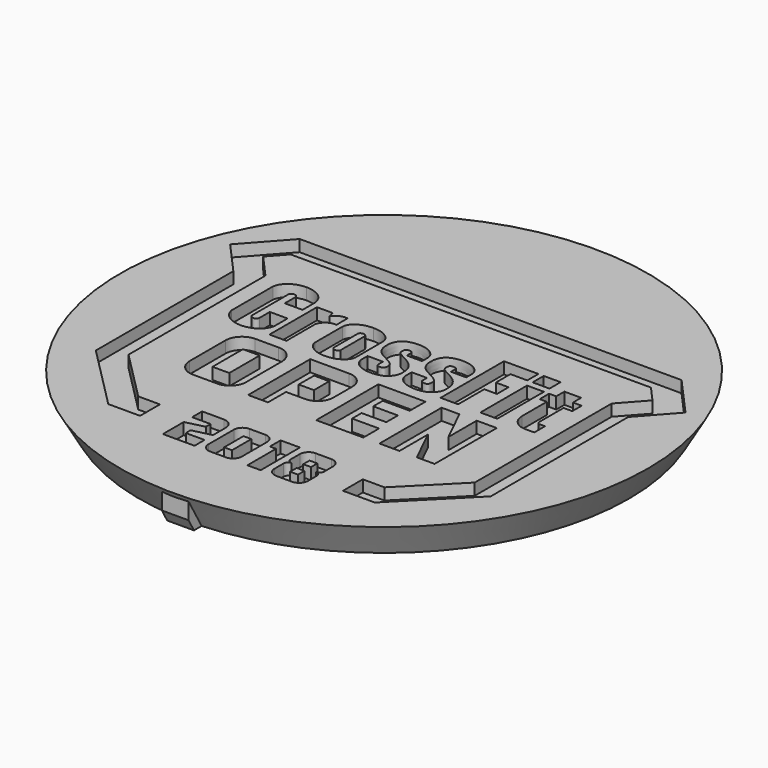
from build123d import *

# Parameters (mm, degrees)
F0_R        = 28.956
F1_DEPTH    = 3.556
F2_W        = 30.4023699468
F2_H        = 2.708328606
F2_W_2      = 1.8437616527
F2_H_2      = 6.3712084666
F2_H_3      = 1.5175901353
F2_W_3      = 1.6611122992
F2_H_4      = 2.0968401222
F2_W_4      = 1.8359664828
F2_H_5      = 4.1484234825
F2_W_5      = 0.8592136437
F2_H_6      = 2.6414245367
F2_H_7      = 0.8889122684
F2_H_8      = 0.8636
F3_DEPTH    = 1.27
F6_DEPTH    = 3.556
F7_T1_DEPTH = 9.4921978168


# Not quite as in the source:
# - a fillet or chamfer that OpenCascade refuses, or shapes differently, is made with other operations: its cross-section is extruded or revolved along the edge and cut away or added


with BuildPart() as f1:
    # F0 (on Top) → F1 (new body)
    with BuildSketch(Plane.XY):
        Circle(F0_R)
    extrude(amount=F1_DEPTH)

    # F2 (on face) → F3 (cut)
    with BuildSketch(Plane.XY.offset(3.556)):
        with Locations((0, 13.1786047998)):
            Rectangle(F2_W, F2_H)
        Polygon((20.8420716974, 14.5327691028), (15.2011849734, 14.5327691028), (15.2011849734, 11.8244404968), (19.6655910583, 11.8244404968), (21.247090707, 10.0590654712), (18.8943144933, 7.4307704384), (18.8943144933, -11.2499324565), (13.4406701729, -16.7418979069), (11.0729235041, -16.7418979069), (11.0729235041, -19.4502265129), (14.5413199249, -19.4502265129), (21.5503721796, -12.3919237413), (21.5503721796, 6.3732514918), (24.849809781, 10.0590654712), align=None)
        Polygon((-15.2011849734, 11.8244404968), (-15.2011849734, 14.5327691028), (-20.8420716974, 14.5327691028), (-24.849809781, 10.0590654712), (-21.5503721796, 6.3732514918), (-21.5503721796, -12.3919237413), (-14.5413199249, -19.4502265129), (-11.0729235041, -19.4502265129), (-11.0729235041, -16.7418979069), (-13.4406701729, -16.7418979069), (-18.8943144933, -11.2499324565), (-18.8943144933, 7.4307704384), (-21.247090707, 10.0590654712), (-19.6655910583, 11.8244404968), align=None)
        with BuildLine():
            ThreePointArc((-15.2091418535, 6.0097032957), (-14.8139919296, 6.2693332665), (-14.4188420058, 6.0097032957))
            Line((-14.4188420058, 6.0097032957), (-14.4188420058, 4.4719388507))
            Line((-14.4188420058, 4.4719388507), (-12.4801692695, 4.4719388507))
            Line((-12.4801692695, 4.4719388507), (-12.4801692695, 6.2930637769))
            add(Edge.make_bspline(
                [(-12.4801692695, 6.2930637769), (-12.5916933403, 6.7707157481), (-12.9251884268, 7.2707731335), (-13.6344023128, 7.7464624472), (-14.2989607428, 7.9362339904), (-14.8139919296, 7.9558056579)],
                knots=[0, 0, 0, 0, 0.3452518733, 0.6338422719, 1, 1, 1, 1], degree=3))
            add(Edge.make_bspline(
                [(-17.1478145898, 6.2930637769), (-17.036290519, 6.7707157481), (-16.7027954325, 7.2707731335), (-15.9935815465, 7.7464624472), (-15.3290231165, 7.9362339904), (-14.8139919296, 7.9558056579)],
                knots=[0, 0, 0, 0, 0.3452518733, 0.6338422719, 1, 1, 1, 1], degree=3))
            Line((-17.1478145898, 6.2930637769), (-17.1478145898, 0.6190669056))
            add(Edge.make_bspline(
                [(-17.1478145898, 0.6190669056), (-17.036290519, 0.1414149345), (-16.7027954325, -0.3586424509), (-15.9935815465, -0.8343317647), (-15.3290231165, -1.0241033079), (-14.8139919296, -1.0436749754)],
                knots=[0, 0, 0, 0, 0.3452518733, 0.6338422719, 1, 1, 1, 1], degree=3))
            add(Edge.make_bspline(
                [(-12.4801692695, 0.6190669056), (-12.5916933403, 0.1414149345), (-12.9251884268, -0.3586424509), (-13.6344023128, -0.8343317647), (-14.2989607428, -1.0241033079), (-14.8139919296, -1.0436749754)],
                knots=[0, 0, 0, 0, 0.3452518733, 0.6338422719, 1, 1, 1, 1], degree=3))
            Line((-12.4801692695, 0.6190669056), (-12.4801692695, 2.4332190197))
            Line((-12.4801692695, 2.4332190197), (-14.4188420058, 2.4332190197))
            Line((-14.4188420058, 2.4332190197), (-14.4188420058, 1.0003426842))
            ThreePointArc((-14.4188420058, 1.0003426842), (-14.8139919296, 0.6797582705), (-15.2091418535, 1.0003426842))
            Line((-15.2091418535, 1.0003426842), (-15.2091418535, 6.0097032957))
        make_face()
        with BuildLine():
            ThreePointArc((-8.498294748, 5.6527445823), (-9.3240459461, 5.52802916), (-9.9700721946, 4.9988136426))
            Line((-9.9700721946, 4.9988136426), (-10.0917066481, 5.6280705877))
            Line((-10.0917066481, 5.6280705877), (-11.8310791474, 5.6280705877))
            Line((-11.8310791474, 5.6280705877), (-11.8310791474, -0.8495571991))
            Line((-11.8310791474, -0.8495571991), (-9.9822352674, -0.8495571991))
            Line((-9.9822352674, -0.8495571991), (-9.9822352674, 3.0987069741))
            ThreePointArc((-9.9822352674, 3.0987069741), (-9.4355214126, 3.8909649876), (-8.498294748, 4.1104529783))
            Line((-8.498294748, 4.1104529783), (-8.498294748, 5.6527445823))
        make_face()
        with BuildLine():
            add(Edge.make_bspline(
                [(-7.8876619975, 4.1982766971), (-7.8356496049, 4.6341372871), (-7.4830251688, 5.0855806361), (-6.6969666534, 5.5265744778), (-6.1764580028, 5.6217318842), (-5.6770178073, 5.6407110794)],
                knots=[0, 0, 0, 0, 0.3397100712, 0.6449265753, 1, 1, 1, 1], degree=3))
            Line((-7.8876619975, 4.1982766971), (-7.8876619975, 0.4633077452))
            add(Edge.make_bspline(
                [(-7.8876619975, 0.4633077452), (-7.8356496049, 0.0274471552), (-7.4830251688, -0.4239961938), (-6.6969666534, -0.8649900355), (-6.1764580028, -0.9601474419), (-5.6770178073, -0.9791266371)],
                knots=[0, 0, 0, 0, 0.3397100712, 0.6449265753, 1, 1, 1, 1], degree=3))
            add(Edge.make_bspline(
                [(-3.4663736171, 0.4633077452), (-3.5183860098, 0.0274471552), (-3.8710104458, -0.4239961938), (-4.6570689612, -0.8649900355), (-5.1775776118, -0.9601474419), (-5.6770178073, -0.9791266371)],
                knots=[0, 0, 0, 0, 0.3397100712, 0.6449265753, 1, 1, 1, 1], degree=3))
            Line((-3.4663736171, 0.4633077452), (-3.4663736171, 4.1982766971))
            add(Edge.make_bspline(
                [(-3.4663736171, 4.1982766971), (-3.5183860098, 4.6341372871), (-3.8710104458, 5.0855806361), (-4.6570689612, 5.5265744778), (-5.1775776118, 5.6217318842), (-5.6770178073, 5.6407110794)],
                knots=[0, 0, 0, 0, 0.3397100712, 0.6449265753, 1, 1, 1, 1], degree=3))
        make_face()
        with BuildLine():
            Line((-6.0537514093, 0.6796154458), (-6.0537514093, 4.0396556988))
            ThreePointArc((-6.0537514093, 4.0396556988), (-5.6770178073, 4.2767262399), (-5.3002842053, 4.0396556988))
            Line((-5.3002842053, 4.0396556988), (-5.3002842053, 0.6796154458))
            ThreePointArc((-5.3002842053, 0.6796154458), (-5.6770178073, 0.4325808427), (-6.0537514093, 0.6796154458))
        make_face(mode=Mode.SUBTRACT)
        with BuildLine():
            add(Edge.make_bspline(
                [(-2.8303159575, 0.3884340668), (-2.8039437057, 0.2035950511), (-2.7084645464, -0.0700189873), (-2.3608920836, -0.4703230086), (-1.9926629718, -0.6996264871), (-1.5028929662, -0.8748491288), (-1.0382407316, -0.9538686812), (-0.6882680471, -0.9546334772), (-0.3368604514, -0.9540527619), (0.2211413136, -0.8513074189), (0.612300795, -0.6901154246), (0.9801185549, -0.3981460143), (1.2267344248, -0.0690546676), (1.3993589582, 0.2977634954), (1.4223729478, 0.7584350911), (1.4049419285, 1.1135593111), (1.3286013981, 1.553696764), (1.1223334914, 1.9521079504), (0.8760135922, 2.2676339155), (0.6015247761, 2.5058684812), (0.2906951276, 2.7053452538), (-0.0001070692, 2.8824823952), (-0.3353974242, 3.0432490404), (-0.5764466432, 3.1792562527), (-0.8154579768, 3.303817088), (-0.9633304165, 3.4276750313), (-1.0959908548, 3.6333141563), (-1.0823984853, 3.8622415727), (-1.0834469924, 4.0754389156), (-0.9485709412, 4.2583690073), (-0.7487440326, 4.3029808765), (-0.5601470729, 4.2949903255), (-0.3773783712, 4.2385764575), (-0.3052749299, 4.1735809243), (-0.2735022713, 4.0681006186)],
                knots=[0, 0, 0, 0, 0.0370250499, 0.0748342879, 0.1100620625, 0.1484988784, 0.1852224027, 0.2162968341, 0.2479903621, 0.2879321478, 0.3230237776, 0.3590762656, 0.3932110531, 0.4269990648, 0.4628119337, 0.4948648069, 0.530192635, 0.5659957163, 0.5996315799, 0.6317213982, 0.6639857771, 0.6953892736, 0.7277821278, 0.7561961656, 0.7835044746, 0.8069782815, 0.8326158776, 0.857980682, 0.8824603672, 0.9067304417, 0.9303429697, 0.953652975, 0.975833924, 1, 1, 1, 1], degree=3))
            Line((-0.2735022713, 4.0681006186), (-0.2735022713, 3.4427449837))
            Line((-0.2735022713, 3.4427449837), (1.3895077923, 3.4427449837))
            Line((1.3895077923, 3.4427449837), (1.3895077923, 4.2547744498))
            add(Edge.make_bspline(
                [(1.3895077923, 4.2547744498), (1.362871865, 4.4414615263), (1.2883734828, 4.7378016949), (0.9605026276, 5.0998324979), (0.5716220009, 5.3815223969), (0.0152610688, 5.5827557819), (-0.3948809767, 5.6297560073), (-0.7047527982, 5.6499225931), (-1.0751777633, 5.6320466323), (-1.6282857111, 5.5504935604), (-2.0336875884, 5.3727640469), (-2.4117723458, 5.0855965451), (-2.6319171142, 4.7457920238), (-2.777638503, 4.3159693257), (-2.7948365878, 3.9652673217), (-2.7867872003, 3.5566089511), (-2.7234512303, 3.1492983197), (-2.4809077804, 2.7167962496), (-2.2560062896, 2.466619706), (-1.9772894721, 2.263975186), (-1.613083499, 2.067015106), (-1.2952433521, 1.9125631017), (-1.0179124703, 1.7567271658), (-0.7490698208, 1.6103729622), (-0.506207899, 1.4077450313), (-0.4071682892, 1.2885965948), (-0.2936071786, 1.0792376552), (-0.3010610885, 0.7910872402), (-0.3213241393, 0.5663172014), (-0.4513056845, 0.4078239751), (-0.6386646385, 0.3709036814), (-0.8427860612, 0.3772912723), (-1.0484772467, 0.4306358217), (-1.1223962588, 0.5223560412), (-1.1560394719, 0.6340462979)],
                knots=[0, 0, 0, 0, 0.0373952344, 0.0734858494, 0.1105806222, 0.1514081281, 0.1855398741, 0.2145930161, 0.246989669, 0.2866513485, 0.3223486125, 0.3583549464, 0.3922575872, 0.4276388924, 0.4592443755, 0.4928782518, 0.5272671439, 0.5643692779, 0.5951310751, 0.6260952205, 0.6604130771, 0.6921960524, 0.7219608284, 0.7518311519, 0.7813056856, 0.8022259164, 0.8274762943, 0.8561110411, 0.8813007038, 0.9041610683, 0.9268832448, 0.9511148768, 0.9744111926, 1, 1, 1, 1], degree=3))
            Line((-1.1560394719, 0.6340462979), (-1.1560394719, 1.2829401795))
            Line((-1.1560394719, 1.2829401795), (-2.8303159575, 1.2829401795))
            Line((-2.8303159575, 1.2829401795), (-2.8303159575, 0.3884340668))
        make_face()
        with BuildLine():
            add(Edge.make_bspline(
                [(1.9797450798, 0.3972758105), (2.0061173315, 0.2124367948), (2.1015964908, -0.0611772436), (2.4491689536, -0.4614812649), (2.8173980654, -0.6907847434), (3.307168071, -0.8660073851), (3.7718203056, -0.9450269375), (4.1217929901, -0.9457917335), (4.4732005858, -0.9452110182), (5.0312023509, -0.8424656752), (5.4223618323, -0.6812736809), (5.7901795921, -0.3893042706), (6.036795462, -0.0602129239), (6.2094199954, 0.3066052391), (6.232433985, 0.7672768348), (6.2150029657, 1.1224010548), (6.1386624353, 1.5625385077), (5.9323945286, 1.9609496941), (5.6860746294, 2.2764756592), (5.4115858133, 2.5147102249), (5.1007561648, 2.7141869975), (4.809953968, 2.8913241389), (4.474663613, 3.0520907841), (4.233614394, 3.1880979964), (3.9946030604, 3.3126588317), (3.8467306207, 3.436516775), (3.7140701824, 3.6421559), (3.7276625519, 3.8710833164), (3.7266140448, 4.0842806593), (3.861490096, 4.267210751), (4.0613170047, 4.3118226202), (4.2499139643, 4.3038320692), (4.4326826661, 4.2474182012), (4.5047861073, 4.182422668), (4.5365587659, 4.0769423623)],
                knots=[0, 0, 0, 0, 0.0370250499, 0.0748342879, 0.1100620625, 0.1484988784, 0.1852224027, 0.2162968341, 0.2479903621, 0.2879321478, 0.3230237776, 0.3590762656, 0.3932110531, 0.4269990648, 0.4628119337, 0.4948648069, 0.530192635, 0.5659957163, 0.5996315799, 0.6317213982, 0.6639857771, 0.6953892736, 0.7277821278, 0.7561961656, 0.7835044746, 0.8069782815, 0.8326158776, 0.857980682, 0.8824603672, 0.9067304417, 0.9303429697, 0.953652975, 0.975833924, 1, 1, 1, 1], degree=3))
            Line((4.5365587659, 4.0769423623), (4.5365587659, 3.4515867274))
            Line((4.5365587659, 3.4515867274), (6.1995688295, 3.4515867274))
            Line((6.1995688295, 3.4515867274), (6.1995688295, 4.2636161935))
            add(Edge.make_bspline(
                [(6.1995688295, 4.2636161935), (6.1729329022, 4.45030327), (6.09843452, 4.7466434386), (5.7705636648, 5.1086742416), (5.3816830381, 5.3903641406), (4.825322106, 5.5915975256), (4.4151800605, 5.638597751), (4.105308239, 5.6587643368), (3.7348832739, 5.640888376), (3.1817753261, 5.5593353041), (2.7763734488, 5.3816057906), (2.3982886914, 5.0944382888), (2.178143923, 4.7546337675), (2.0324225342, 4.3248110694), (2.0152244495, 3.9741090653), (2.0232738369, 3.5654506948), (2.0866098069, 3.1581400634), (2.3291532568, 2.7256379933), (2.5540547477, 2.4754614497), (2.8327715651, 2.2728169297), (3.1969775382, 2.0758568497), (3.5148176851, 1.9214048454), (3.7921485669, 1.7655689095), (4.0609912164, 1.6192147059), (4.3038531382, 1.416586775), (4.402892748, 1.2974383385), (4.5164538586, 1.0880793989), (4.5089999487, 0.7999289839), (4.4887368979, 0.5751589451), (4.3587553528, 0.4166657188), (4.1713963987, 0.3797454251), (3.967274976, 0.386133016), (3.7615837905, 0.4394775654), (3.6876647784, 0.5311977848), (3.6540215653, 0.6428880416)],
                knots=[0, 0, 0, 0, 0.0373952344, 0.0734858494, 0.1105806222, 0.1514081281, 0.1855398741, 0.2145930161, 0.246989669, 0.2866513485, 0.3223486125, 0.3583549464, 0.3922575872, 0.4276388924, 0.4592443755, 0.4928782518, 0.5272671439, 0.5643692779, 0.5951310751, 0.6260952205, 0.6604130771, 0.6921960524, 0.7219608284, 0.7518311519, 0.7813056856, 0.8022259164, 0.8274762943, 0.8561110411, 0.8813007038, 0.9041610683, 0.9268832448, 0.9511148768, 0.9744111926, 1, 1, 1, 1], degree=3))
            Line((3.6540215653, 0.6428880416), (3.6540215653, 1.2917819232))
            Line((3.6540215653, 1.2917819232), (1.9797450798, 1.2917819232))
            Line((1.9797450798, 1.2917819232), (1.9797450798, 0.3972758105))
        make_face()
        Polygon((10.6105204249, 6.2751232445), (10.6105204249, 7.7927133799), (6.8492461505, 7.7927133799), (6.8492461505, -0.854884015), (8.7667587722, -0.854884015), (8.7667587722, 2.7055770889), (10.1574822838, 2.7055770889), (10.1574822838, 4.2872906461), (8.7667587722, 4.2872906461), (8.7667587722, 6.2751232445), align=None)
        with Locations((12.1124403237, 2.3307202183)):
            Rectangle(F2_W_2, F2_H_2)
        with Locations((12.1124403237, 7.0339183122)):
            Rectangle(F2_W_2, F2_H_3)
        with BuildLine():
            Line((16.2016264889, 6.6334225968), (14.3765285406, 6.6334225968))
            Line((14.3765285406, 6.6334225968), (14.3765285406, 5.5163244516))
            Line((14.3765285406, 5.5163244516), (13.5945966262, 5.5163244516))
            Line((13.5945966262, 5.5163244516), (13.5945966262, 4.2304804347))
            Line((13.5945966262, 4.2304804347), (14.3765285406, 4.2304804347))
            Line((14.3765285406, 4.2304804347), (14.3765285406, 0.8540854588))
            ThreePointArc((14.3765285406, 0.8540854588), (14.8770741106, -0.354338445), (16.0854980144, -0.854884015))
            Line((16.0854980144, -0.854884015), (17.0765723828, -0.854884015))
            Line((17.0765723828, -0.854884015), (17.0765723828, 0.6118975844))
            Line((17.0765723828, 0.6118975844), (16.5136363152, 0.6118975844))
            ThreePointArc((16.5136363152, 0.6118975844), (16.2930120512, 0.7032831468), (16.2016264889, 0.9239074107))
            Line((16.2016264889, 0.9239074107), (16.2016264889, 4.2304804347))
            Line((16.2016264889, 4.2304804347), (17.1537883374, 4.2304804347))
            Line((17.1537883374, 4.2304804347), (17.1537883374, 5.5163244516))
            Line((17.1537883374, 5.5163244516), (16.2016264889, 5.5163244516))
            Line((16.2016264889, 5.5163244516), (16.2016264889, 6.6334225968))
        make_face()
        Polygon((9.9929075049, -2.2195314625), (8.0549451523, -2.2195314625), (8.0549451523, -10.6973991598), (10.2406190708, -10.6973991598), (10.2406190708, -6.8355969954), (12.134869583, -10.6973991598), (14.0728319356, -10.6973991598), (14.0728319356, -2.2195314625), (11.887158017, -2.2195314625), (11.887158017, -6.0813336269), align=None)
        Polygon((6.2918351032, -2.2195314625), (1.148215495, -2.2195314625), (1.148215495, -10.6973991598), (6.2918351032, -10.6973991598), (6.2918351032, -8.5553083438), (3.3484606538, -8.5553083438), (3.3484606538, -7.2576974643), (6.0441256501, -7.2576974643), (6.0441256501, -5.6740386746), (3.3484606538, -5.659233158), (3.3484606538, -4.3616222785), (6.2918351032, -4.3616222785), align=None)
        with BuildLine():
            Line((-2.0720108878, -2.2195314625), (-6.28307648, -2.2195314625))
            Line((-6.28307648, -2.2195314625), (-6.28307648, -10.6973991598))
            Line((-6.28307648, -10.6973991598), (-4.1119735688, -10.6973991598))
            Line((-4.1119735688, -10.6973991598), (-4.1119735688, -8.2385173984))
            Line((-4.1119735688, -8.2385173984), (-2.0720108878, -8.2385173984))
            ThreePointArc((-2.0720108878, -8.2385173984), (-0.8289668197, -7.7600961181), (-0.3089004895, -6.5338920205))
            Line((-0.3089004895, -6.5338920205), (-0.3089004895, -3.9241568404))
            ThreePointArc((-0.3089004895, -3.9241568404), (-0.8289668197, -2.6979527428), (-2.0720108878, -2.2195314625))
        make_face()
        with Locations((-3.2959884265, -5.4402171329)):
            Rectangle(F2_W_3, F2_H_4, mode=Mode.SUBTRACT)
        with BuildLine():
            ThreePointArc((-12.3009653762, -2.2195314625), (-13.5702499026, -2.7657857878), (-14.0932183713, -4.0448405081))
            Line((-14.0932183713, -4.0448405081), (-14.0932183713, -8.9475232046))
            ThreePointArc((-14.0932183713, -8.9475232046), (-13.5533866968, -10.1873844568), (-12.3009653762, -10.6973991598))
            Line((-12.3009653762, -10.6973991598), (-9.7364410758, -10.6973991598))
            ThreePointArc((-9.7364410758, -10.6973991598), (-8.443681983, -10.2156752838), (-7.900474593, -8.9475232046))
            Line((-7.900474593, -8.9475232046), (-7.900474593, -4.0448405081))
            ThreePointArc((-7.900474593, -4.0448405081), (-8.4419792148, -2.7535092189), (-9.7364410758, -2.2195314625))
            Line((-9.7364410758, -2.2195314625), (-12.3009653762, -2.2195314625))
        make_face()
        with Locations((-10.9895607457, -6.4509226824)):
            Rectangle(F2_W_4, F2_H_5, mode=Mode.SUBTRACT)
        with BuildLine():
            ThreePointArc((-3.9980014447, -16.5996085636), (-4.3188053633, -15.8251193924), (-5.0932945345, -15.5043154738))
            Line((-5.0932945345, -15.5043154738), (-7.4532657057, -15.5043154738))
            Line((-7.4532657057, -15.5043154738), (-7.4532657057, -16.8733258668))
            Line((-7.4532657057, -16.8733258668), (-5.4378226526, -16.8733258668))
            Line((-5.4378226526, -16.8733258668), (-5.4378226526, -17.5226714457))
            Line((-5.4378226526, -17.5226714457), (-7.4532657057, -18.0188127658))
            Line((-7.4532657057, -18.0188127658), (-7.4532657057, -20.862694544))
            Line((-7.4532657057, -20.862694544), (-3.9980014447, -20.862694544))
            Line((-3.9980014447, -20.862694544), (-3.9980014447, -19.493684151))
            Line((-3.9980014447, -19.493684151), (-6.0480448617, -19.493684151))
            Line((-6.0480448617, -19.493684151), (-6.0480448617, -18.8443385721))
            Line((-6.0480448617, -18.8443385721), (-3.9980014447, -18.3396796855))
            Line((-3.9980014447, -18.3396796855), (-3.9980014447, -16.5996085636))
        make_face()
        with BuildLine():
            Line((-0.556260686, -15.5043154738), (-2.2857946936, -15.5043154738))
            ThreePointArc((-2.2857946936, -15.5043154738), (-2.9607040326, -15.7838720754), (-3.2402606342, -16.4587814144))
            Line((-3.2402606342, -16.4587814144), (-3.2402606342, -19.9082286034))
            ThreePointArc((-3.2402606342, -19.9082286034), (-2.9607040326, -20.5831379424), (-2.2857946936, -20.862694544))
            Line((-2.2857946936, -20.862694544), (-0.556260686, -20.862694544))
            ThreePointArc((-0.556260686, -20.862694544), (0.118648653, -20.5831379424), (0.3982052546, -19.9082286034))
            Line((0.3982052546, -19.9082286034), (0.3982052546, -16.4587814144))
            ThreePointArc((0.3982052546, -16.4587814144), (0.118648653, -15.7838720754), (-0.556260686, -15.5043154738))
        make_face()
        with Locations((-1.418305725, -18.1940381352)):
            Rectangle(F2_W_5, F2_H_6, mode=Mode.SUBTRACT)
        Polygon((3.2210330352, -15.5043154738), (1.1077687483, -15.5043154738), (1.1077687483, -16.9665754709), (1.7710558711, -16.9665754709), (1.7710558711, -20.862694544), (3.2210330352, -20.862694544), align=None)
        with BuildLine():
            ThreePointArc((7.6090606342, -16.4587814144), (7.3295040326, -15.7838720754), (6.6545946936, -15.5043154738))
            Line((6.6545946936, -15.5043154738), (4.925060686, -15.5043154738))
            ThreePointArc((4.925060686, -15.5043154738), (4.250151347, -15.7838720754), (3.9705947454, -16.4587814144))
            Line((3.9705947454, -16.4587814144), (3.9705947454, -17.7062390089))
            ThreePointArc((3.9705947454, -17.7062390089), (4.1103827204, -18.0437170339), (4.4478607454, -18.1835050089))
            ThreePointArc((4.4478607454, -18.1835050089), (4.1103827204, -18.3232929839), (3.9705947454, -18.6607710089))
            Line((3.9705947454, -18.6607710089), (3.9705947454, -19.9082286034))
            ThreePointArc((3.9705947454, -19.9082286034), (4.250151347, -20.5831379424), (4.925060686, -20.862694544))
            Line((4.925060686, -20.862694544), (6.6545946936, -20.862694544))
            ThreePointArc((6.6545946936, -20.862694544), (7.3295040326, -20.5831379424), (7.6090606342, -19.9082286034))
            Line((7.6090606342, -19.9082286034), (7.6090606342, -18.6607710089))
            ThreePointArc((7.6090606342, -18.6607710089), (7.4692726592, -18.3232929839), (7.1317946342, -18.1835050089))
            ThreePointArc((7.1317946342, -18.1835050089), (7.4692726592, -18.0437170339), (7.6090606342, -17.7062390089))
            Line((7.6090606342, -17.7062390089), (7.6090606342, -16.4587814144))
        make_face()
        with Locations((5.787105725, -19.0702942693)):
            Rectangle(F2_W_5, F2_H_7, mode=Mode.SUBTRACT)
        with Locations((5.787105725, -17.3051258668)):
            Rectangle(F2_W_5, F2_H_8, mode=Mode.SUBTRACT)
    extrude(amount=-F3_DEPTH, mode=Mode.SUBTRACT)

    # F4: chamfer of 3.81 x 2.1997045256 on 1 edges, made by hand

    # F4_s1 → F4_t2 (revolve, cut)
    with BuildSketch(Plane.XZ):
        Polygon((28.956, 3.81), (26.7562954744, 0), (28.956, 0), align=None)
    revolve(axis=Axis((0, 0, 0), (0, 0, 1)), mode=Mode.SUBTRACT)

    # F5 (on face) → F6 (join, through all)
    with BuildSketch(Plane.XY.offset(3.556)):
        with BuildLine():
            ThreePointArc((1.4605, -26.7164048342), (0, -26.7562954744), (-1.4605, -26.7164048342))
            Line((-1.4605, -26.7164048342), (-1.4605, -28.4944048342))
            Line((-1.4605, -28.4944048342), (1.4605, -28.4944048342))
            Line((1.4605, -28.4944048342), (1.4605, -26.7164048342))
        make_face()
    extrude(amount=-F6_DEPTH)

    # F7: chamfer of 1.27 x 0.7332348419 on 1 edges, made by hand

    # F7_s2 → F7_t1 (cut)
    with BuildSketch(Plane.YZ.offset(-4.7460989084)):
        Polygon((-27.7611699923, 0), (-28.4944048342, 1.27), (-28.4944048342, 0), align=None)
    extrude(amount=F7_T1_DEPTH, mode=Mode.SUBTRACT)


solid = f1.part
